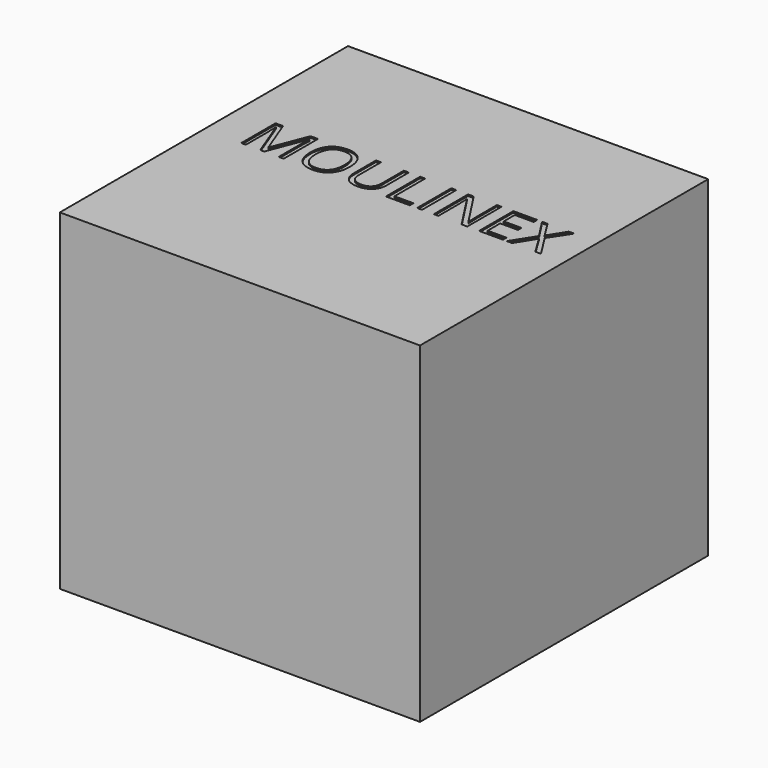
from build123d import *

# Parameters (mm, degrees)
F0_W         = 250
F0_H         = 250
F1_DEPTH     = 230
F2_TEXT_SIZE = 41.6666666667
F3_DEPTH     = 1


# Not quite as in the source:
# - Text() gives the source's letters only with a copy of the font that has no kerning and outlines rounded to 1/6400 em; it was checked with that copy


with BuildPart() as f1:
    # F0 (on Top) → F1 (new body)
    with BuildSketch(Plane.XY):
        Rectangle(F0_W, F0_H)
    extrude(amount=F1_DEPTH)

    # F2 (on face) → F3 (cut)
    with BuildSketch(Plane.XY.offset(230)):
        with Locations((-103.1697881367, 0)):
            Text('MOULINEX', F2_TEXT_SIZE, font='Open Sans', text_align=(TextAlign.LEFT, TextAlign.BOTTOM))
    extrude(amount=-F3_DEPTH, mode=Mode.SUBTRACT)


solid = f1.part
